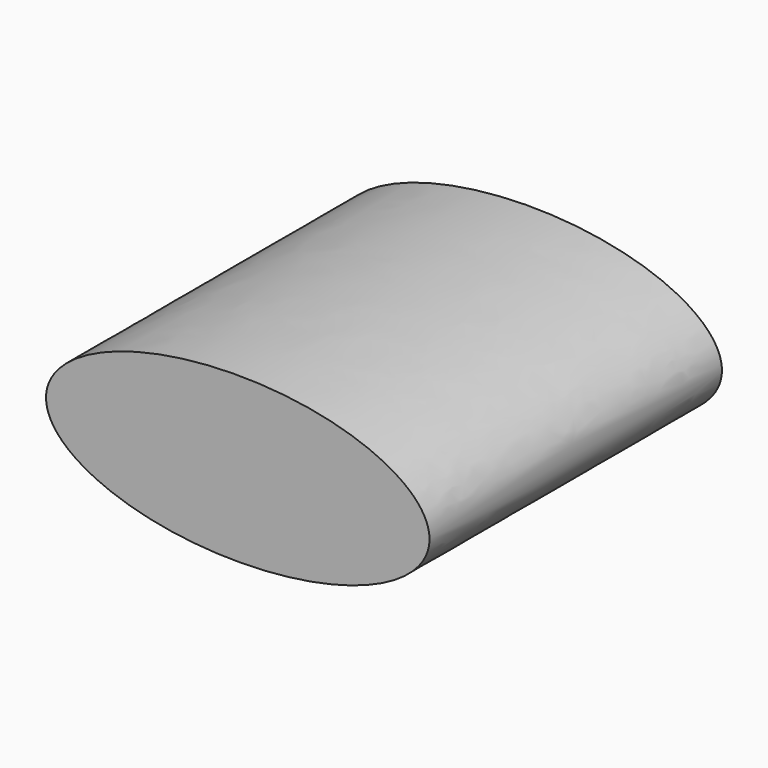
from build123d import *

# Parameters (mm, degrees)
F0_R     = 11.6941232586
F0_R_2   = 7.942283416
F1_DEPTH = 101.6


with BuildPart() as f1:
    # F0 (on Front) → F1 (new body)
    with BuildSketch(Plane.XZ):
        with BuildLine():
            add(Edge.make_bspline(
                [(53.2885119319, 0), (53.2885119319, 39.5160869482), (-26.6442559659, 19.7580434741), (-106.5770238638, 0), (-26.6442559659, -19.7580434741), (53.2885119319, -39.5160869482), (53.2885119319, 0)],
                knots=[0, 0, 0, 2.0943951024, 2.0943951024, 4.1887902048, 4.1887902048, 6.2831853072, 6.2831853072, 6.2831853072], degree=2, weights=[1, 0.5, 1, 0.5, 1, 0.5, 1]))
        make_face()
        with Locations((-22.7055419236, 0)):
            Circle(F0_R, mode=Mode.SUBTRACT)
        with Locations((20.2341880649, 0)):
            Circle(F0_R_2, mode=Mode.SUBTRACT)
        with Locations((-22.7055419236, 0)):
            Circle(F0_R)
        with Locations((20.2341880649, 0)):
            Circle(F0_R_2)
    extrude(amount=F1_DEPTH)


solid = f1.part
